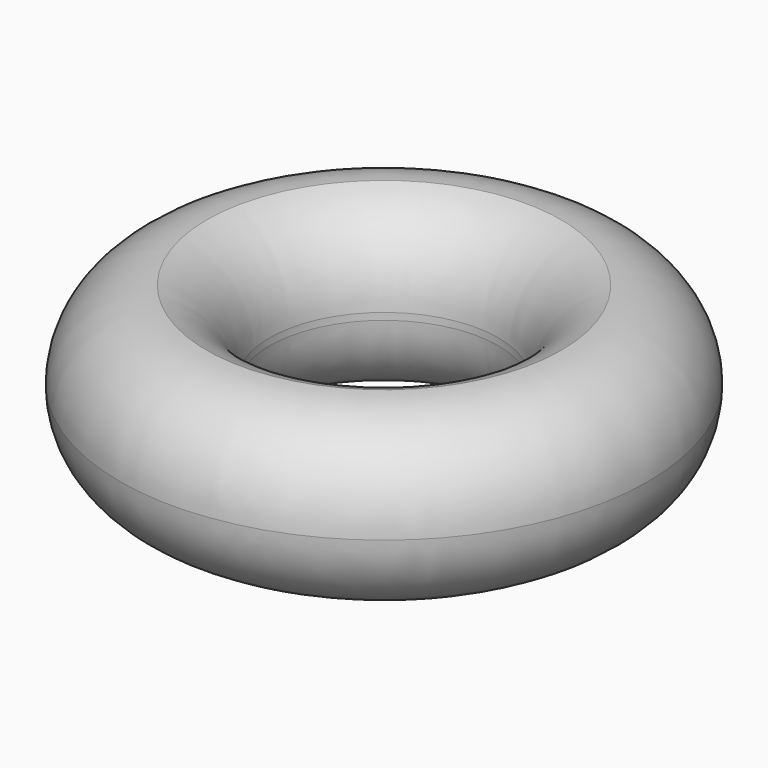
from build123d import *

# Parameters (mm, degrees)
F0_R     = 38.5379103623
F0_R_2   = 16.6938076384
F1_DEPTH = 25.4
F2_R     = 12.69999


# Not quite as in the source:
# - a fillet or chamfer that OpenCascade refuses, or shapes differently, is made with other operations: its cross-section is extruded or revolved along the edge and cut away or added
# - a fillet or chamfer is up to 0.001 mm smaller than in the source, because OpenCascade refuses the exact size


with BuildPart() as f1:
    # F0 (on Top) → F1 (new body)
    with BuildSketch(Plane.XY):
        Circle(F0_R)
        Circle(F0_R_2, mode=Mode.SUBTRACT)
    extrude(amount=F1_DEPTH)

    # F2 (radius 12.7 in the source; OpenCascade refuses exactly that, so slightly less here)
    f2_edges = [f1.edges().sort_by_distance(p)[0] for p in [
        (-38.53791, 0, 25.4),
        (-38.53791, 0, 0),
    ]]
    fillet(f2_edges, radius=F2_R)

    # F3: fillet of radius 12.7 on 2 edges, made by hand

    # F3_s1 → F3_t2 (revolve, cut)
    with BuildSketch(Plane.XZ):
        with BuildLine():
            ThreePointArc((25.8379203623, 25.4), (19.2338428647, 20.8280140909), (16.6938076384, 13.2079671228))
            Line((16.6938076384, 13.2079671228), (16.6938076384, 25.4))
            Line((16.6938076384, 25.4), (25.8379203623, 25.4))
        make_face()
    revolve(axis=Axis((0, 0, 25.4), (0, 0, 1)), mode=Mode.SUBTRACT)

    # F3_s3 → F3_t4 (revolve, cut)
    with BuildSketch(Plane.XZ):
        with BuildLine():
            ThreePointArc((25.8379203623, 0), (19.2338428647, 4.5719859091), (16.6938076384, 12.1920328772))
            Line((16.6938076384, 12.1920328772), (16.6938076384, 0))
            Line((16.6938076384, 0), (25.8379203623, 0))
        make_face()
    revolve(axis=Axis((0, 0, 0), (0, 0, 1)), mode=Mode.SUBTRACT)


solid = f1.part
